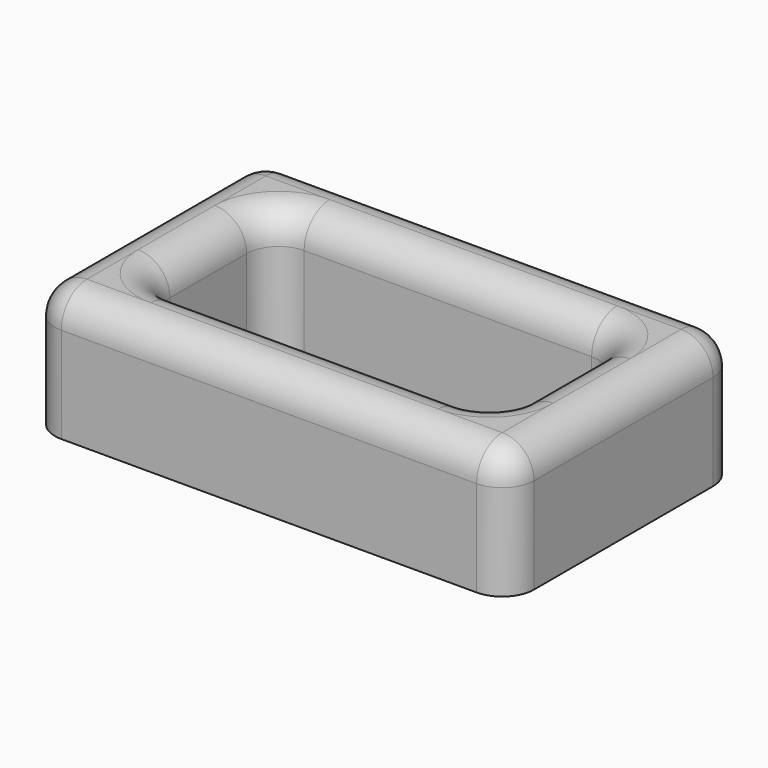
from build123d import *

# Parameters (mm, degrees)
F0_W     = 15
F0_H     = 9
F0_W_2   = 11
F0_H_2   = 5
F1_DEPTH = 4
F2_R     = 0.99999


# Not quite as in the source:
# - a fillet or chamfer is up to 0.001 mm smaller than in the source, because OpenCascade refuses the exact size


with BuildPart() as f1:
    # F0 (on Top) → F1 (new body)
    with BuildSketch(Plane.XY):
        with Locations((5.5, 2.5)):
            Rectangle(F0_W, F0_H)
        with Locations((5.5, 2.5)):
            Rectangle(F0_W_2, F0_H_2, mode=Mode.SUBTRACT)
    extrude(amount=F1_DEPTH)

    # F2 (radius 1 in the source; OpenCascade refuses exactly that, so slightly less here)
    f2_edges = [f1.edges().sort_by_distance(p)[0] for p in [
        (5.5, -2, 4),
        (13, 2.5, 4),
        (5.5, 0, 4),
        (-2, 2.5, 4),
        (0, 2.5, 4),
        (5.5, 7, 4),
        (5.5, 5, 4),
        (11, 2.5, 4),
        (-2, -2, 2),
        (13, -2, 2),
        (11, 0, 2),
        (0, 0, 2),
        (-2, 7, 2),
        (13, 7, 2),
        (11, 5, 2),
        (0, 5, 2),
    ]]
    fillet(f2_edges, radius=F2_R)


solid = f1.part
